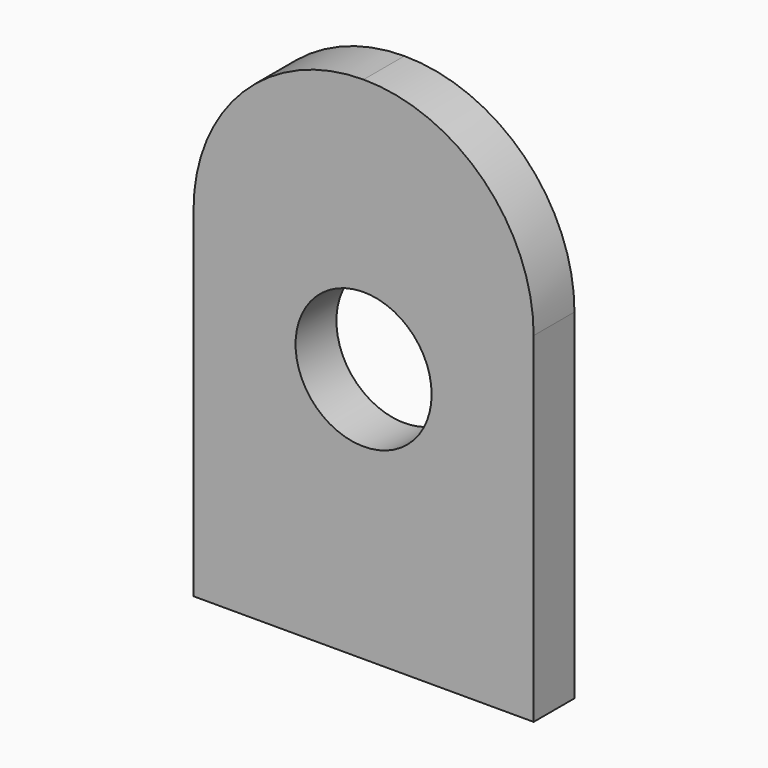
from build123d import *

# Parameters (mm, degrees)
F0_W     = 20
F0_H     = 30
F0_R     = 4
F1_DEPTH = 3
F2_R     = 9.99999


# Not quite as in the source:
# - a fillet or chamfer is up to 0.001 mm smaller than in the source, because OpenCascade refuses the exact size


with BuildPart() as f1:
    # F0 (on Front) → F1 (new body)
    with BuildSketch(Plane.XZ):
        with Locations((10, 15)):
            Rectangle(F0_W, F0_H)
        with Locations((10, 15)):
            Circle(F0_R, mode=Mode.SUBTRACT)
    extrude(amount=F1_DEPTH)

    # F2 (radius 10 in the source; OpenCascade refuses exactly that, so slightly less here)
    f2_edges = [f1.edges().sort_by_distance(p)[0] for p in [
        (0, -1.5, 30),
        (20, -1.5, 30),
    ]]
    fillet(f2_edges, radius=F2_R)


solid = f1.part
